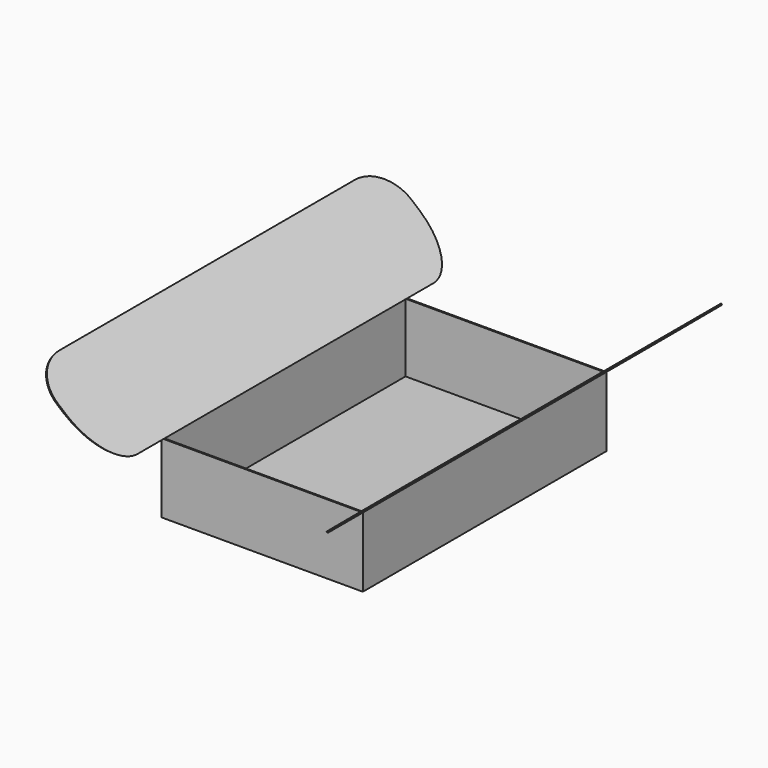
from build123d import *

# Parameters (mm, degrees)
F0_W         = 390
F0_H         = 135
F1_DEPTH     = 590
F2_W         = 384.5905684095
F2_H         = 585
F3_DEPTH     = 132.5
F5_DEPTH     = 590
F7_DEPTH     = 133
F8_T1_DEPTH  = 352.5
F8_T3_DEPTH  = 353.8893095672
F8_T5_DEPTH  = 353.8893095672
F8_T7_DEPTH  = 352.5
F10_DEPTH    = 133
F11_T1_DEPTH = 352.5
F11_T3_DEPTH = 353.8893095672
F11_T5_DEPTH = 353.8893095672
F11_T7_DEPTH = 352.5


# Not quite as in the source:
# - a fillet or chamfer that OpenCascade refuses, or shapes differently, is made with other operations: its cross-section is extruded or revolved along the edge and cut away or added


with BuildPart() as f1:
    # F0 (on Front) → F1 (new body)
    with BuildSketch(Plane.XZ):
        Rectangle(F0_W, F0_H)
    extrude(amount=-F1_DEPTH)

    # F2 (on face) → F3 (cut)
    with BuildSketch(Plane.XY.offset(67.5)):
        with Locations((0, 295)):
            Rectangle(F2_W, F2_H)
    extrude(amount=-F3_DEPTH, mode=Mode.SUBTRACT)

    # F4 (on face) → F5 (join)
    with BuildSketch(Plane.XZ):
        Polygon((-195, 67.5), (-191.1106904328, 67.5), (-342.771697384, 194.7586949967), (-344.3786664082, 192.8435838889), align=None)
        Polygon((191.1106904328, 67.5), (195, 67.5), (344.3786664082, 192.8435838889), (342.771697384, 194.7586949967), align=None)
    extrude(amount=-F5_DEPTH)

    # F6 (on face) → F7 (join)
    with BuildSketch(Plane(origin=(0, 590, 0), x_dir=(-1, 0, 0), z_dir=(0, 1, 0))):
        Polygon((195, 67.5), (344.3786664082, 192.8435838889), (342.771697384, 194.7586949967), (191.1106904328, 67.5), align=None)
        Polygon((-344.3786664082, 192.8435838889), (-195, 67.5), (-191.1106904328, 67.5), (-342.771697384, 194.7586949967), align=None)
    extrude(amount=F7_DEPTH)

    # F8: fillet of radius 70 on 4 edges, made by hand

    # F8_s2 → F8_t1 (cut)
    with BuildSketch(Plane(origin=(-66.762759706, 0, 79.5647587312), x_dir=(0, 1, 0), z_dir=(0.6427876097, 0, -0.7660444431))):
        with BuildLine():
            ThreePointArc((723, 317.766830062), (702.4974746831, 367.2643047451), (653, 387.766830062))
            Line((653, 387.766830062), (723, 387.766830062))
            Line((723, 387.766830062), (723, 317.766830062))
        make_face()
    extrude(amount=F8_T1_DEPTH, mode=Mode.SUBTRACT)

    # F8_s4 → F8_t3 (cut)
    with BuildSketch(Plane.YZ.offset(16.1106904328)):
        with BuildLine():
            ThreePointArc((653, 67.5), (702.4974746831, 88.0025253169), (723, 137.5))
            Line((723, 137.5), (723, 67.5))
            Line((723, 67.5), (653, 67.5))
        make_face()
    extrude(amount=F8_T3_DEPTH, mode=Mode.SUBTRACT)

    # F8_s6 → F8_t5 (cut)
    with BuildSketch(Plane.YZ.offset(-370)):
        with BuildLine():
            ThreePointArc((723, 137.5), (702.4974746831, 88.0025253169), (653, 67.5))
            Line((653, 67.5), (723, 67.5))
            Line((723, 67.5), (723, 137.5))
        make_face()
    extrude(amount=F8_T5_DEPTH, mode=Mode.SUBTRACT)

    # F8_s8 → F8_t7 (cut)
    with BuildSketch(Plane(origin=(-159.8198727085, 0, -190.4659074683), x_dir=(0, 1, 0), z_dir=(0.6427876097, 0, 0.7660444431))):
        with BuildLine():
            ThreePointArc((653, 387.766830062), (702.4974746831, 367.2643047451), (723, 317.766830062))
            Line((723, 317.766830062), (723, 387.766830062))
            Line((723, 387.766830062), (653, 387.766830062))
        make_face()
    extrude(amount=F8_T7_DEPTH, mode=Mode.SUBTRACT)

    # F9 (on face) → F10 (join)
    with BuildSketch(Plane.XZ):
        Polygon((342.771697384, 194.7586949967), (191.1106904328, 67.5), (195, 67.5), (344.3786664082, 192.8435838889), align=None)
        Polygon((-195, 67.5), (-191.1106904328, 67.5), (-342.771697384, 194.7586949967), (-344.3786664082, 192.8435838889), align=None)
    extrude(amount=F10_DEPTH)

    # F11: fillet of radius 70 on 4 edges, made by hand

    # F11_s2 → F11_t1 (cut)
    with BuildSketch(Plane(origin=(66.762759706, 0, 79.5647587312), x_dir=(0, 1, 0), z_dir=(-0.6427876097, 0, -0.7660444431))):
        with BuildLine():
            ThreePointArc((-63, -387.766830062), (-112.4974746831, -367.2643047451), (-133, -317.766830062))
            Line((-133, -317.766830062), (-133, -387.766830062))
            Line((-133, -387.766830062), (-63, -387.766830062))
        make_face()
    extrude(amount=F11_T1_DEPTH, mode=Mode.SUBTRACT)

    # F11_s4 → F11_t3 (cut)
    with BuildSketch(Plane.YZ.offset(-370)):
        with BuildLine():
            ThreePointArc((-133, 137.5), (-112.4974746831, 88.0025253169), (-63, 67.5))
            Line((-63, 67.5), (-133, 67.5))
            Line((-133, 67.5), (-133, 137.5))
        make_face()
    extrude(amount=F11_T3_DEPTH, mode=Mode.SUBTRACT)

    # F11_s6 → F11_t5 (cut)
    with BuildSketch(Plane.YZ.offset(16.1106904328)):
        with BuildLine():
            ThreePointArc((-63, 67.5), (-112.4974746831, 88.0025253169), (-133, 137.5))
            Line((-133, 137.5), (-133, 67.5))
            Line((-133, 67.5), (-63, 67.5))
        make_face()
    extrude(amount=F11_T5_DEPTH, mode=Mode.SUBTRACT)

    # F11_s8 → F11_t7 (cut)
    with BuildSketch(Plane(origin=(159.8198727085, 0, -190.4659074683), x_dir=(0, 1, 0), z_dir=(-0.6427876097, 0, 0.7660444431))):
        with BuildLine():
            ThreePointArc((-133, -317.766830062), (-112.4974746831, -367.2643047451), (-63, -387.766830062))
            Line((-63, -387.766830062), (-133, -387.766830062))
            Line((-133, -387.766830062), (-133, -317.766830062))
        make_face()
    extrude(amount=F11_T7_DEPTH, mode=Mode.SUBTRACT)


solid = f1.part
